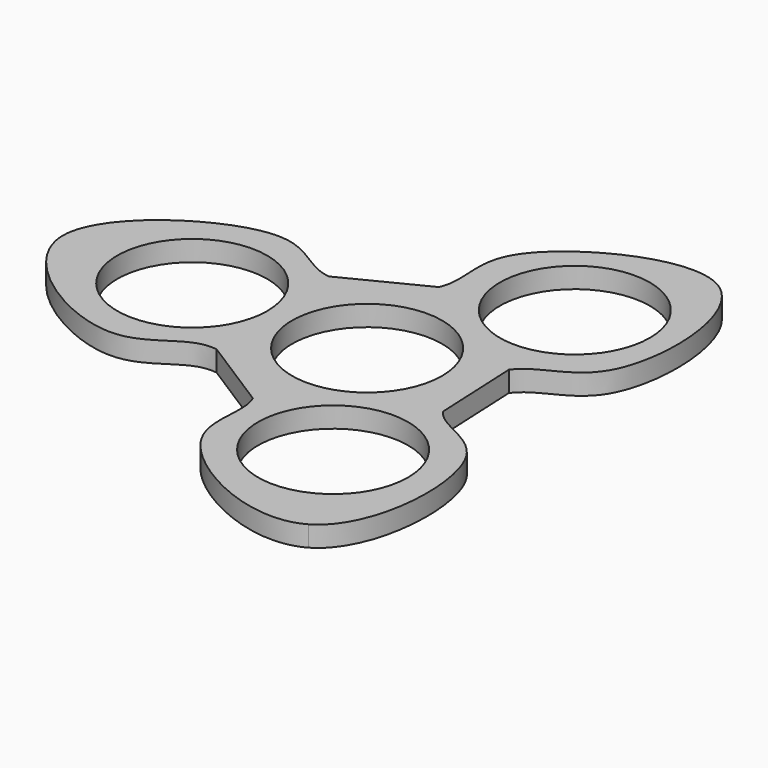
from build123d import *

# Parameters (mm, degrees)
F0_R     = 10.95
F1_DEPTH = 3


with BuildPart() as f1:
    # F0 (on Top) → F1 (new body)
    with BuildSketch(Plane.XY):
        with BuildLine():
            add(Edge.make_bspline(
                [(-5.8011541485, 13.4066559206), (-8.8676045727, 12.2590908018), (-11.8929318418, 10.8319905852), (-14.3401725667, 11.0545409956)],
                knots=[0.1249323841, 0.1249323841, 0.1249323841, 0.1249323841, 0.3163146937, 0.3163146937, 0.3163146937, 0.3163146937], degree=3))
            add(Edge.make_bspline(
                [(-14.3401725667, 11.0545409956), (-17.8866489744, 11.377055153), (-23.6363273691, 20.7122598252), (-44.3589256829, 7.4970639444), (-44.3427115679, 0)],
                knots=[0.3163146937, 0.3163146937, 0.3163146937, 0.3163146937, 0.5936608654, 1, 1, 1, 1], degree=3))
            add(Edge.make_bspline(
                [(-13.1242937512, -10.9792726354), (-13.6173826323, -10.9196115122), (-17.7715627839, -10.7977766057), (-23.5877063126, -20.776971945), (-44.358917025, -7.4930607147), (-44.3427115679, 0)],
                knots=[0.2829494547, 0.2829494547, 0.2829494547, 0.2829494547, 0.3185350392, 0.5938778395, 1, 1, 1, 1], degree=3))
            add(Edge.make_bspline(
                [(-7.0715763163, -12.9002769191), (-9.2053325351, -12.0583537713), (-11.2872682999, -11.2015429116), (-13.1242937512, -10.9792726354)],
                knots=[0.1503737125, 0.1503737125, 0.1503737125, 0.1503737125, 0.2829494547, 0.2829494547, 0.2829494547, 0.2829494547], degree=3))
            add(Edge.make_bspline(
                [(-7.0715763163, -12.9002769191), (-5.0421401822, -14.5132693334), (-3.1401674186, -16.0847991906), (-2.3396282292, -17.8476460659)],
                knots=[0.1675183718, 0.1675183718, 0.1675183718, 0.1675183718, 0.3185350392, 0.3185350392, 0.3185350392, 0.3185350392], degree=3))
            add(Edge.make_bspline(
                [(-2.3396282292, -17.8476460659), (-0.880036345, -21.0617760252), (-6.3296277169, -30.5907081208), (15.5601822262, -41.9371486499), (22.0412604287, -38.1765839551)],
                knots=[0.3185350392, 0.3185350392, 0.3185350392, 0.3185350392, 0.5938778395, 1, 1, 1, 1], degree=3))
            add(Edge.make_bspline(
                [(16.6263281137, -6.8976460659), (18.6800503675, -9.7687546964), (29.6571433192, -9.8137361759), (28.5385440883, -34.4440879352), (22.0412604287, -38.1765839551)],
                knots=[0.3185350392, 0.3185350392, 0.3185350392, 0.3185350392, 0.5938778395, 1, 1, 1, 1], degree=3))
            add(Edge.make_bspline(
                [(14.4529803487, 1.3727601674), (14.944518042, -1.7812527521), (15.2528202178, -4.9774787372), (16.6263281137, -6.8976460659)],
                knots=[0.1343886633, 0.1343886633, 0.1343886633, 0.1343886633, 0.3185350392, 0.3185350392, 0.3185350392, 0.3185350392], degree=3))
            add(Edge.make_bspline(
                [(14.4529803487, 1.3727601674), (14.7789199493, 3.1398634963), (15.2190111691, 4.7329381595), (16.0357763561, 5.8747778475)],
                knots=[0.2090312281, 0.2090312281, 0.2090312281, 0.2090312281, 0.3185350392, 0.3185350392, 0.3185350392, 0.3185350392], degree=3))
            add(Edge.make_bspline(
                [(16.0357763561, 5.8747778475), (18.0894986098, 8.7458864781), (29.0665915616, 8.7908679575), (27.9479923307, 33.4212197169), (21.4507086711, 37.1537157367)],
                knots=[0.3185350392, 0.3185350392, 0.3185350392, 0.3185350392, 0.5938778395, 1, 1, 1, 1], degree=3))
            add(Edge.make_bspline(
                [(-2.9301799868, 16.8247778475), (-1.4705881026, 20.0389078069), (-6.9201794745, 29.5678399025), (14.9696304686, 40.9142804316), (21.4507086711, 37.1537157367)],
                knots=[0.3185350392, 0.3185350392, 0.3185350392, 0.3185350392, 0.5938778395, 1, 1, 1, 1], degree=3))
            add(Edge.make_bspline(
                [(-5.8011541485, 13.4066559206), (-4.537281533, 14.5062302906), (-3.4768859657, 15.6208905932), (-2.9301799868, 16.8247778475)],
                knots=[0.2154024055, 0.2154024055, 0.2154024055, 0.2154024055, 0.3185350392, 0.3185350392, 0.3185350392, 0.3185350392], degree=3))
        make_face()
        with Locations((12.732138116, -22.0527101059)):
            Circle(F0_R, mode=Mode.SUBTRACT)
        with Locations((-25.464276232, 0)):
            Circle(F0_R, mode=Mode.SUBTRACT)
        with Locations((0.1072884321, -0.0640614032)):
            Circle(F0_R, mode=Mode.SUBTRACT)
        with Locations((12.732138116, 22.0527101059)):
            Circle(F0_R, mode=Mode.SUBTRACT)
        with BuildLine():
            Line((-2.9301799868, 16.8247778475), (-14.3401725667, 11.0545409956))
            add(Edge.make_bspline(
                [(-5.8011541485, 13.4066559206), (-8.8676045727, 12.2590908018), (-11.8929318418, 10.8319905852), (-14.3401725667, 11.0545409956)],
                knots=[0.1249323841, 0.1249323841, 0.1249323841, 0.1249323841, 0.3163146937, 0.3163146937, 0.3163146937, 0.3163146937], degree=3))
            add(Edge.make_bspline(
                [(-5.8011541485, 13.4066559206), (-4.537281533, 14.5062302906), (-3.4768859657, 15.6208905932), (-2.9301799868, 16.8247778475)],
                knots=[0.2154024055, 0.2154024055, 0.2154024055, 0.2154024055, 0.3185350392, 0.3185350392, 0.3185350392, 0.3185350392], degree=3))
        make_face()
        with BuildLine():
            add(Edge.make_bspline(
                [(-7.0715763163, -12.9002769191), (-9.2053325351, -12.0583537713), (-11.2872682999, -11.2015429116), (-13.1242937512, -10.9792726354)],
                knots=[0.1503737125, 0.1503737125, 0.1503737125, 0.1503737125, 0.2829494547, 0.2829494547, 0.2829494547, 0.2829494547], degree=3))
            Line((-13.1242937512, -10.9792726354), (-2.3396282292, -17.8476460657))
            add(Edge.make_bspline(
                [(-7.0715763163, -12.9002769191), (-5.0421401822, -14.5132693334), (-3.1401674186, -16.0847991906), (-2.3396282292, -17.8476460659)],
                knots=[0.1675183718, 0.1675183718, 0.1675183718, 0.1675183718, 0.3185350392, 0.3185350392, 0.3185350392, 0.3185350392], degree=3))
        make_face()
        with BuildLine():
            Line((16.6263281137, -6.8976460659), (16.035776356, 5.8747778474))
            add(Edge.make_bspline(
                [(14.4529803487, 1.3727601674), (14.7789199493, 3.1398634963), (15.2190111691, 4.7329381595), (16.0357763561, 5.8747778475)],
                knots=[0.2090312281, 0.2090312281, 0.2090312281, 0.2090312281, 0.3185350392, 0.3185350392, 0.3185350392, 0.3185350392], degree=3))
            add(Edge.make_bspline(
                [(14.4529803487, 1.3727601674), (14.944518042, -1.7812527521), (15.2528202178, -4.9774787372), (16.6263281137, -6.8976460659)],
                knots=[0.1343886633, 0.1343886633, 0.1343886633, 0.1343886633, 0.3185350392, 0.3185350392, 0.3185350392, 0.3185350392], degree=3))
        make_face()
    extrude(amount=F1_DEPTH)


solid = f1.part
